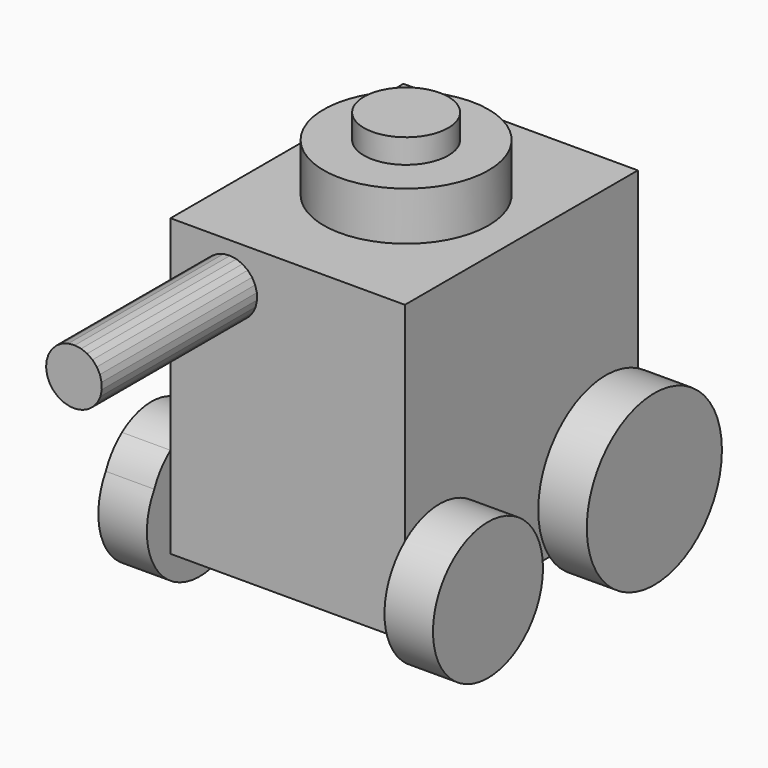
from build123d import *

# Parameters (mm, degrees)
F1_DEPTH  = 25.4
F2_DEPTH  = 127
F3_W      = 122.7013282478
F3_H      = 129.251409322
F4_DEPTH  = 76.2
F5_DEPTH  = 76.2
F6_DEPTH  = 25.4
F7_R      = 35.9848930873
F8_DEPTH  = 25.4
F9_R      = 44.2111783383
F10_DEPTH = 25.4
F13_R     = 34.5791946556
F12_R     = 32.2271478821
F14_DEPTH = 25.4
F15_R     = 43.299097817
F16_DEPTH = 25.4
F17_R     = 43.1496203252
F18_DEPTH = 25.4
F19_R     = 22.0921612012
F20_DEPTH = 12.7
F21_R     = 45.7423711287
F22_DEPTH = 7.62
F23_DEPTH = 25.4


# Not quite as in the source:
# - a feature names something its author has since deleted; it is built from what else it names


with BuildPart() as f1:
    # F0 (on Front) → F1 (new body)
    with BuildSketch(Plane.XZ):
        Polygon((-46.2158193521, 37.6598188143), (-45.7216948271, 34.3051441014), (-44.4672482626, 31.1548480371), (-42.5201071978, 28.3787638977), (-39.9852425112, 26.1265510978), (-36.9993094144, 24.5196270122), (-33.7232803334, 23.6446213344), (-30.333766844, 23.548705847), (-27.0134984958, 24.2370513787), (-23.9414718147, 25.6725490438), (-21.2833005544, 27.7778107915), (-19.1822874155, 30.4393414161), (-17.7516985602, 33.5136571128), (-17.068657404, 36.8350207265), (-17.1699868723, 40.2243766851), (-18.0502242674, 43.4990039316), (-19.6619157634, 46.4823664636), (-21.9181746546, 49.0136304347), (-24.6973654401, 50.9563347491), (-27.8496612254, 52.2057477143), (-31.2051209287, 52.6945131539), (-34.5828508489, 52.3962815967), (-37.8007566917, 51.3271307829), (-40.6853603202, 49.5446989099), (-43.0811520061, 47.1450773411), (-44.8589739995, 44.2576302965), (-45.9229834566, 41.0380207937), align=None)
    extrude(amount=F1_DEPTH)

    # F2 (add): a face of the model
    f2_faces = [f1.faces().sort_by_distance(p)[0] for p in [
        (-31.618218869, -25.4, 38.0962342024),
    ]]
    extrude(f2_faces, amount=F2_DEPTH)

    # F3 (on Front) → F4 (join)
    with BuildSketch(Plane.XZ):
        with Locations((-1.0198447853, -4.8156213015)):
            Rectangle(F3_W, F3_H)
    extrude(amount=F4_DEPTH)

    # F5 (add): a face of the model
    f5_faces = [f1.faces().sort_by_distance(p)[0] for p in [
        (-1.0198447853, 0, -4.8156213015),
    ]]
    extrude(f5_faces, amount=F5_DEPTH)

    # F6 (add): a face of the model
    f6_faces = [f1.faces().sort_by_distance(p)[0] for p in [
        (-1.0198447853, 0, -69.4413259625),
    ]]
    extrude(f6_faces, amount=F6_DEPTH)

    # F7 (on face) → F8 (join)
    with BuildSketch(Plane.YZ.offset(60.3308193386)):
        with Locations((-53.5847470164, -77.124491334)):
            Circle(F7_R)
    extrude(amount=F8_DEPTH)

    # F9 (on face) → F10 (join)
    with BuildSketch(Plane.YZ.offset(60.3308193386)):
        with Locations((55.2663691342, -70.2658891678)):
            Circle(F9_R)
    extrude(amount=F10_DEPTH)

    # F13 (on face) + F12 (on face) → F14 (join)
    with BuildSketch(Plane(origin=(-62.3705089092, 0, 0), x_dir=(0, -1, 0), z_dir=(-1, 0, 0))):
        with Locations((57.0854917169, -78.4721449018)):
            Circle(F13_R)
    with BuildSketch(Plane(origin=(-62.3705089092, 0, 0), x_dir=(0, -1, 0), z_dir=(-1, 0, 0))):
        with Locations((56.974042207, -73.0006918311)):
            Circle(F12_R)
        with BuildLine():
            Line((76.2, -94.8413259625), (76.2, -47.1365930153))
            ThreePointArc((76.2, -47.1365930153), (33.0171171216, -51.4448387729), (33.2764524277, -94.8413259625))
            Line((33.2764524277, -94.8413259625), (76.2, -94.8413259625))
        make_face()
    extrude(amount=F14_DEPTH)

    # F15 (on face) → F16 (join)
    with BuildSketch(Plane(origin=(-62.3705089092, 0, 0), x_dir=(0, -1, 0), z_dir=(-1, 0, 0))):
        with Locations((-55.8602996171, -70.3753679991)):
            Circle(F15_R)
    extrude(amount=F16_DEPTH)

    # F17 (on face) → F18 (join)
    with BuildSketch(Plane.XY.offset(59.8100833595)):
        Circle(F17_R)
    extrude(amount=F18_DEPTH)

    # F19 (on face) → F20 (join)
    with BuildSketch(Plane.XY.offset(85.2100833595)):
        Circle(F19_R)
    extrude(amount=F20_DEPTH)

    # F21 (on face) → F22 (join)
    with BuildSketch(Plane(origin=(0, 76.2, 0), x_dir=(-1, 0, 0), z_dir=(0, 1, 0))):
        with Locations((0, -36.8642732501)):
            Circle(F21_R)
    extrude(amount=F22_DEPTH)

    # F23 (add): a face of the model
    f23_faces = [f1.faces().sort_by_distance(p)[0] for p in [
        (-31.618218869, -152.4, 38.0962342024),
    ]]
    extrude(f23_faces, amount=F23_DEPTH)


solid = f1.part
